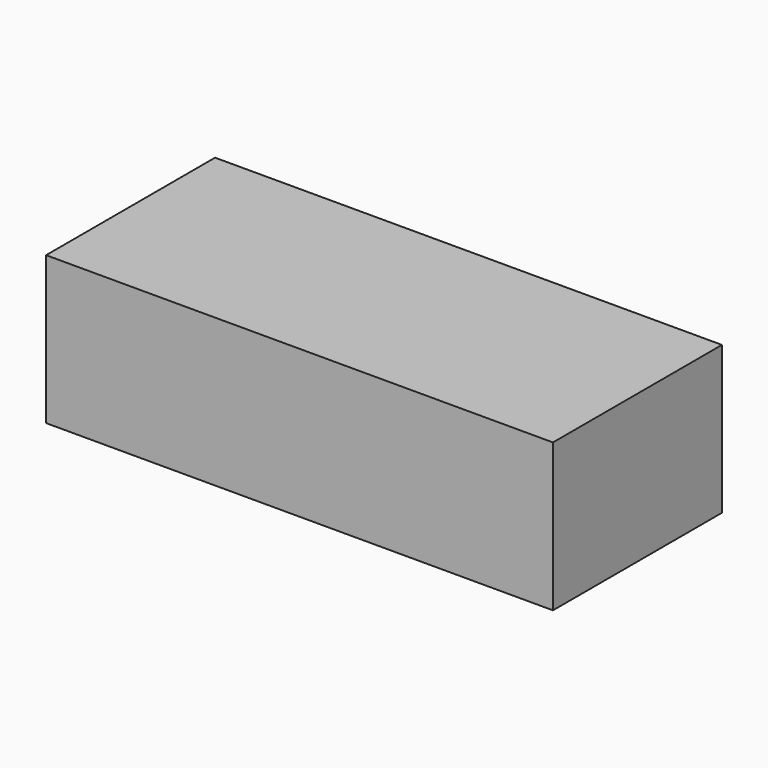
from build123d import *

# Parameters (mm, degrees)
F0_W     = 50
F0_H     = 35
F1_DEPTH = 60


# Not quite as in the source:
# - a feature of the source that left no trace in its solid (it failed there, or was rolled back) is left out


with BuildPart() as f1:
    # F0 (on Right) → F1 (new body, symmetric)
    with BuildSketch(Plane.YZ):
        with Locations((-60, -22.5)):
            Rectangle(F0_W, F0_H)
    extrude(amount=F1_DEPTH, both=True)


solid = f1.part
